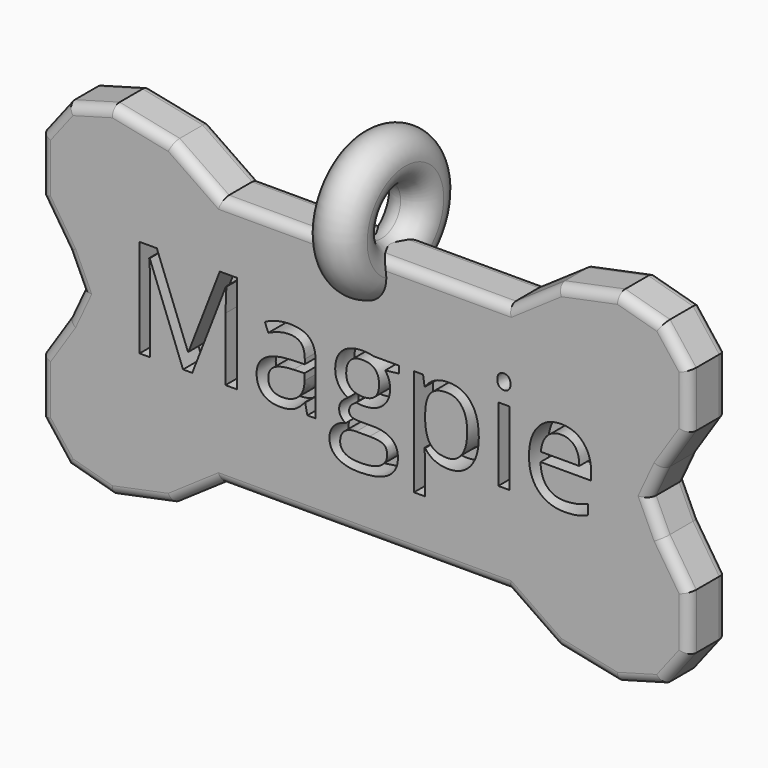
from build123d import *

# Parameters (mm, degrees)
F1_DEPTH     = 2.54
F2_R         = 0.508
F3_TEXT_SIZE = 7.3108556939
F4_DEPTH     = 1.27


# Not quite as in the source:
# - Text() gives the source's letters only with a copy of the font that has no kerning and outlines rounded to 1/6400 em; it was checked with that copy


with BuildPart() as f1:
    # F0 (on Front) → F1 (new body)
    with BuildSketch(Plane.XZ):
        Polygon((2.0103843274, 6.6693559441), (-5.6096156726, 6.6693559441), (-13.2296156726, 6.6693559441), (-15.8515510253, 8.4719367156), (-19.0470352022, 9.127420742), (-21.4231646474, 8.4719367156), (-22.8160668483, 6.6693559441), (-22.8160668483, 3.7196781265), (-21.4231646474, 1.5893559441), (-20.6857440637, 0), (-21.4231646474, -1.5893559441), (-22.8160668483, -3.7196781265), (-22.8160668483, -6.6693559441), (-21.4231646474, -8.4719367156), (-19.0470352022, -9.127420742), (-15.8515510253, -8.4719367156), (-13.2296156726, -6.6693559441), (-5.6096156726, -6.6693559441), (2.0103843274, -6.6693559441), (4.6323196802, -8.4719367156), (7.8278038571, -9.127420742), (10.2039333023, -8.4719367156), (11.5968355032, -6.6693559441), (11.5968355032, -3.7196781265), (10.2039333023, -1.5893559441), (9.4665127186, 0), (10.2039333023, 1.5893559441), (11.5968355032, 3.7196781265), (11.5968355032, 6.6693559441), (10.2039333023, 8.4719367156), (7.8278038571, 9.127420742), (4.6323196802, 8.4719367156), align=None)
    extrude(amount=F1_DEPTH)

    # F2
    f2_edges = [f1.edges().sort_by_distance(p)[0] for p in [
        (6.230062, -2.54, 8.799679),
        (3.321352, -2.54, 7.570646),
        (-5.609616, -2.54, 6.669356),
        (-14.540583, -2.54, 7.570646),
        (-17.449293, -2.54, 8.799679),
        (-20.2351, -2.54, 8.799679),
        (-22.119616, -2.54, 7.570646),
        (-22.816067, -2.54, 5.194517),
        (-22.119616, -2.54, 2.654517),
        (-21.054454, -2.54, 0.794678),
        (-21.054454, -2.54, -0.794678),
        (-22.119616, -2.54, -2.654517),
        (-22.816067, -2.54, -5.194517),
        (-22.119616, -2.54, -7.570646),
        (-20.2351, -2.54, -8.799679),
        (-17.449293, -2.54, -8.799679),
        (-14.540583, -2.54, -7.570646),
        (-5.609616, -2.54, -6.669356),
        (3.321352, -2.54, -7.570646),
        (6.230062, -2.54, -8.799679),
        (9.015869, -2.54, -8.799679),
        (10.900384, -2.54, -7.570646),
        (11.596836, -2.54, -5.194517),
        (10.900384, -2.54, -2.654517),
        (9.835223, -2.54, -0.794678),
        (9.835223, -2.54, 0.794678),
        (10.900384, -2.54, 2.654517),
        (11.596836, -2.54, 5.194517),
        (10.900384, -2.54, 7.570646),
        (9.015869, -2.54, 8.799679),
        (6.230062, 0, 8.799679),
        (3.321352, 0, 7.570646),
        (-5.609616, 0, 6.669356),
        (-14.540583, 0, 7.570646),
        (-17.449293, 0, 8.799679),
        (-20.2351, 0, 8.799679),
        (-22.119616, 0, 7.570646),
        (-22.816067, 0, 5.194517),
        (-22.119616, 0, 2.654517),
        (-21.054454, 0, 0.794678),
        (-21.054454, 0, -0.794678),
        (-22.119616, 0, -2.654517),
        (-22.816067, 0, -5.194517),
        (-22.119616, 0, -7.570646),
        (-20.2351, 0, -8.799679),
        (-17.449293, 0, -8.799679),
        (-14.540583, 0, -7.570646),
        (-5.609616, 0, -6.669356),
        (3.321352, 0, -7.570646),
        (6.230062, 0, -8.799679),
        (9.015869, 0, -8.799679),
        (10.900384, 0, -7.570646),
        (11.596836, 0, -5.194517),
        (10.900384, 0, -2.654517),
        (9.835223, 0, -0.794678),
        (9.835223, 0, 0.794678),
        (10.900384, 0, 2.654517),
        (11.596836, 0, 5.194517),
        (10.900384, 0, 7.570646),
        (9.015869, 0, 8.799679),
    ]]
    fillet(f2_edges, radius=F2_R)

    # F3 (on face) → F4 (cut)
    with BuildSketch(Plane.XZ.offset(2.54)):
        with Locations((-18.2996690273, -1.9462750643)):
            Text('Magpie', F3_TEXT_SIZE, font='Open Sans', text_align=(TextAlign.LEFT, TextAlign.BOTTOM))
    extrude(amount=-F4_DEPTH, mode=Mode.SUBTRACT)

    # F6 (on offset) → F7 (revolve)
    with BuildSketch(Plane.XZ.offset(1.27)):
        with BuildLine():
            ThreePointArc((-5.7404, 6.7623230782), (-6.6384256121, 4.5942974661), (-4.4704, 5.4923230782))
            ThreePointArc((-4.4704, 5.4923230782), (-4.8423743879, 6.3903486903), (-5.7404, 6.7623230782))
        make_face()
    revolve(axis=Axis((-2.6754314768, -1.27, 8.0323230782), (1, 0, 0)))


solid = f1.part
